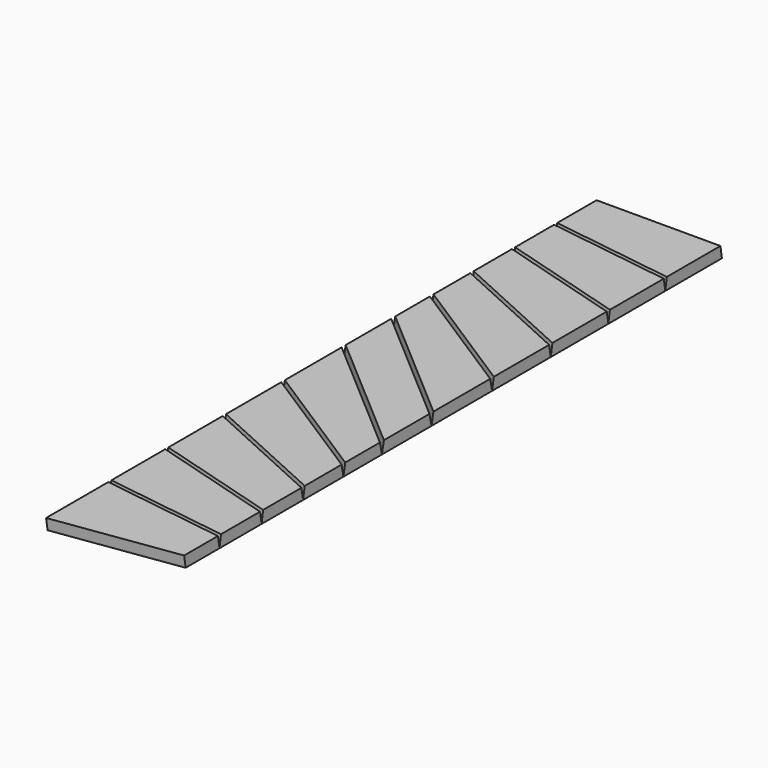
from build123d import *

# Parameters (mm, degrees)
F2_DEPTH    = 9.525
F3_DEPTH    = 9.525
F4_DEPTH    = 9.525
F5_DEPTH    = 9.525
F6_DEPTH    = 9.525
F7_DEPTH    = 9.525
F8_DEPTH    = 9.525
F9_DEPTH    = 9.525
F10_DEPTH   = 9.525
F11_DEPTH   = 9.525
F12_DEPTH   = 9.525
F13_SIZE2   = 1.550911
F13_SIZE    = 9.52499
F13_2_SIZE2 = 1.550911
F13_2_SIZE  = 9.52499
F14_SIZE2   = 1.550911
F14_SIZE    = 9.52499
F14_2_SIZE2 = 1.550911
F14_2_SIZE  = 9.52499
F15_SIZE2   = 1.550911
F15_SIZE    = 9.52499
F15_2_SIZE2 = 1.550911
F15_2_SIZE  = 9.52499
F16_SIZE2   = 1.550911
F16_SIZE    = 9.52499
F16_2_SIZE2 = 1.550911
F16_2_SIZE  = 9.52499
F17_SIZE2   = 1.550911
F17_SIZE    = 9.52499
F17_2_SIZE2 = 1.550911
F17_2_SIZE  = 9.52499
F18_SIZE2   = 1.550911
F18_SIZE    = 9.52499
F18_2_SIZE2 = 1.550911
F18_2_SIZE  = 9.52499
F19_SIZE2   = 1.550911
F19_SIZE    = 9.52499
F19_2_SIZE2 = 1.550911
F19_2_SIZE  = 9.52499
F20_SIZE2   = 1.550911
F20_SIZE    = 9.52499
F20_2_SIZE2 = 1.550911
F20_2_SIZE  = 9.52499
F21_SIZE2   = 1.550911
F21_SIZE    = 9.52499
F21_2_SIZE2 = 1.550911
F21_2_SIZE  = 9.52499
F22_SIZE2   = 1.550911
F22_SIZE    = 9.52499
F22_2_SIZE2 = 1.550911
F22_2_SIZE  = 9.52499
F23_SIZE2   = 1.550911
F23_SIZE    = 9.52499
F24_SIZE2   = 1.550911
F24_SIZE    = 9.52499


# Not quite as in the source:
# - a fillet or chamfer is up to 0.001 mm smaller than in the source, because OpenCascade refuses the exact size


with BuildPart() as f2:
    # F1 (on Top) → F2 (new body)
    with BuildSketch(Plane.XY):
        Polygon((50.8, 279.4), (-50.8, 279.4), (-50.8, 235.8864560812), (50.8, 221.3135439188), align=None)
    extrude(amount=F2_DEPTH)

    # F13 (size 9.525 and 1.5509205186 in the source; OpenCascade refuses exactly that, so slightly less here)
    f13_edges = [f2.edges().sort_by_distance(p)[0] for p in [
        (0, 228.6, 9.525),
    ]]
    f13_side = f2.faces().sort_by_distance((0, 228.6, 4.7625))[0]
    chamfer(f13_edges, length=F13_SIZE, length2=F13_SIZE2, reference=f13_side)

    # F13#2 (size 9.525 and 1.5509205186 in the source; OpenCascade refuses exactly that, so slightly less here)
    f13_2_edges = [f2.edges().sort_by_distance(p)[0] for p in [
        (0, 279.4, 9.525),
    ]]
    f13_2_side = f2.faces().sort_by_distance((0, 279.4, 4.7625))[0]
    chamfer(f13_2_edges, length=F13_2_SIZE, length2=F13_2_SIZE2, reference=f13_2_side)


with BuildPart() as f3:
    # F1 (on Top) → F3 (new body)
    with BuildSketch(Plane.XY):
        Polygon((50.8, 221.3135439188), (-50.8, 235.8864560812), (-50.8, 192.6790237109), (50.8, 162.9209762891), align=None)
    extrude(amount=F3_DEPTH)

    # F14 (size 9.525 and 1.5509205186 in the source; OpenCascade refuses exactly that, so slightly less here)
    f14_edges = [f3.edges().sort_by_distance(p)[0] for p in [
        (0, 228.6, 9.525),
    ]]
    f14_side = f3.faces().sort_by_distance((0, 228.6, 4.7625))[0]
    chamfer(f14_edges, length=F14_SIZE, length2=F14_SIZE2, reference=f14_side)

    # F14#2 (size 9.525 and 1.5509205186 in the source; OpenCascade refuses exactly that, so slightly less here)
    f14_2_edges = [f3.edges().sort_by_distance(p)[0] for p in [
        (0, 177.8, 9.525),
    ]]
    f14_2_side = f3.faces().sort_by_distance((0, 177.8, 4.7625))[0]
    chamfer(f14_2_edges, length=F14_2_SIZE, length2=F14_2_SIZE2, reference=f14_2_side)


with BuildPart() as f4:
    # F1 (on Top) → F4 (new body)
    with BuildSketch(Plane.XY):
        Polygon((50.8, 162.9209762891), (-50.8, 192.6790237109), (-50.8, 150.1375105152), (50.8, 103.8624894848), align=None)
    extrude(amount=F4_DEPTH)

    # F15 (size 9.525 and 1.5509205186 in the source; OpenCascade refuses exactly that, so slightly less here)
    f15_edges = [f4.edges().sort_by_distance(p)[0] for p in [
        (0, 177.8, 9.525),
    ]]
    f15_side = f4.faces().sort_by_distance((0, 177.8, 4.7625))[0]
    chamfer(f15_edges, length=F15_SIZE, length2=F15_SIZE2, reference=f15_side)

    # F15#2 (size 9.525 and 1.5509205186 in the source; OpenCascade refuses exactly that, so slightly less here)
    f15_2_edges = [f4.edges().sort_by_distance(p)[0] for p in [
        (0, 127, 9.525),
    ]]
    f15_2_side = f4.faces().sort_by_distance((0, 127, 4.7625))[0]
    chamfer(f15_2_edges, length=F15_2_SIZE, length2=F15_2_SIZE2, reference=f15_2_side)


with BuildPart() as f5:
    # F1 (on Top) → F5 (new body)
    with BuildSketch(Plane.XY):
        Polygon((50.8, 103.8624894848), (-50.8, 150.1375105152), (-50.8, 108.75045291), (50.8, 43.64954709), align=None)
    extrude(amount=F5_DEPTH)

    # F16 (size 9.525 and 1.5509205186 in the source; OpenCascade refuses exactly that, so slightly less here)
    f16_edges = [f5.edges().sort_by_distance(p)[0] for p in [
        (0, 127, 9.525),
    ]]
    f16_side = f5.faces().sort_by_distance((0, 127, 4.7625))[0]
    chamfer(f16_edges, length=F16_SIZE, length2=F16_SIZE2, reference=f16_side)

    # F16#2 (size 9.525 and 1.5509205186 in the source; OpenCascade refuses exactly that, so slightly less here)
    f16_2_edges = [f5.edges().sort_by_distance(p)[0] for p in [
        (0, 76.2, 9.525),
    ]]
    f16_2_side = f5.faces().sort_by_distance((0, 76.2, 4.7625))[0]
    chamfer(f16_2_edges, length=F16_2_SIZE, length2=F16_2_SIZE2, reference=f16_2_side)


with BuildPart() as f6:
    # F1 (on Top) → F6 (new body)
    with BuildSketch(Plane.XY):
        Polygon((50.8, 43.64954709), (-50.8, 108.75045291), (-50.8, 69.2687277608), (50.8, -18.4687277608), align=None)
    extrude(amount=F6_DEPTH)

    # F17 (size 9.525 and 1.5509205186 in the source; OpenCascade refuses exactly that, so slightly less here)
    f17_edges = [f6.edges().sort_by_distance(p)[0] for p in [
        (0, 25.4, 9.525),
    ]]
    f17_side = f6.faces().sort_by_distance((0, 25.4, 4.7625))[0]
    chamfer(f17_edges, length=F17_SIZE, length2=F17_SIZE2, reference=f17_side)

    # F17#2 (size 9.525 and 1.5509205186 in the source; OpenCascade refuses exactly that, so slightly less here)
    f17_2_edges = [f6.edges().sort_by_distance(p)[0] for p in [
        (0, 76.2, 9.525),
    ]]
    f17_2_side = f6.faces().sort_by_distance((0, 76.2, 4.7625))[0]
    chamfer(f17_2_edges, length=F17_2_SIZE, length2=F17_2_SIZE2, reference=f17_2_side)


with BuildPart() as f7:
    # F1 (on Top) → F7 (new body)
    with BuildSketch(Plane.XY):
        Polygon((50.8, -18.4687277608), (-50.8, 69.2687277608), (-50.8, 18.4687277609), (50.7999999999, -69.2687277608), align=None)
    extrude(amount=F7_DEPTH)

    # F18 (size 9.525 and 1.5509205186 in the source; OpenCascade refuses exactly that, so slightly less here)
    f18_edges = [f7.edges().sort_by_distance(p)[0] for p in [
        (0, 25.4, 9.525),
    ]]
    f18_side = f7.faces().sort_by_distance((0, 25.4, 4.7625))[0]
    chamfer(f18_edges, length=F18_SIZE, length2=F18_SIZE2, reference=f18_side)

    # F18#2 (size 9.525 and 1.5509205186 in the source; OpenCascade refuses exactly that, so slightly less here)
    f18_2_edges = [f7.edges().sort_by_distance(p)[0] for p in [
        (0, -25.4, 9.525),
    ]]
    f18_2_side = f7.faces().sort_by_distance((0, -25.4, 4.7625))[0]
    chamfer(f18_2_edges, length=F18_2_SIZE, length2=F18_2_SIZE2, reference=f18_2_side)


with BuildPart() as f8:
    # F1 (on Top) → F8 (new body)
    with BuildSketch(Plane.XY):
        Polygon((50.7999999999, -69.2687277608), (-50.8000000001, 18.4687277609), (-50.8, -43.64954709), (50.7999999999, -108.7504529099), align=None)
    extrude(amount=F8_DEPTH)

    # F19 (size 9.525 and 1.5509205186 in the source; OpenCascade refuses exactly that, so slightly less here)
    f19_edges = [f8.edges().sort_by_distance(p)[0] for p in [
        (0, -25.4, 9.525),
    ]]
    f19_side = f8.faces().sort_by_distance((0, -25.4, 4.7625))[0]
    chamfer(f19_edges, length=F19_SIZE, length2=F19_SIZE2, reference=f19_side)

    # F19#2 (size 9.525 and 1.5509205186 in the source; OpenCascade refuses exactly that, so slightly less here)
    f19_2_edges = [f8.edges().sort_by_distance(p)[0] for p in [
        (0, -76.2, 9.525),
    ]]
    f19_2_side = f8.faces().sort_by_distance((0, -76.2, 4.7625))[0]
    chamfer(f19_2_edges, length=F19_2_SIZE, length2=F19_2_SIZE2, reference=f19_2_side)


with BuildPart() as f9:
    # F1 (on Top) → F9 (new body)
    with BuildSketch(Plane.XY):
        Polygon((50.7999999999, -108.7504529099), (-50.8000000001, -43.64954709), (-50.8, -103.8624894848), (50.7999999999, -150.1375105152), align=None)
    extrude(amount=F9_DEPTH)

    # F20 (size 9.525 and 1.5509205186 in the source; OpenCascade refuses exactly that, so slightly less here)
    f20_edges = [f9.edges().sort_by_distance(p)[0] for p in [
        (0, -76.2, 9.525),
    ]]
    f20_side = f9.faces().sort_by_distance((0, -76.2, 4.7625))[0]
    chamfer(f20_edges, length=F20_SIZE, length2=F20_SIZE2, reference=f20_side)

    # F20#2 (size 9.525 and 1.5509205186 in the source; OpenCascade refuses exactly that, so slightly less here)
    f20_2_edges = [f9.edges().sort_by_distance(p)[0] for p in [
        (0, -127, 9.525),
    ]]
    f20_2_side = f9.faces().sort_by_distance((0, -127, 4.7625))[0]
    chamfer(f20_2_edges, length=F20_2_SIZE, length2=F20_2_SIZE2, reference=f20_2_side)


with BuildPart() as f10:
    # F1 (on Top) → F10 (new body)
    with BuildSketch(Plane.XY):
        Polygon((50.7999999999, -150.1375105152), (-50.8000000001, -103.8624894848), (-50.8, -162.9209762891), (50.7999999999, -192.6790237109), align=None)
    extrude(amount=F10_DEPTH)

    # F21 (size 9.525 and 1.5509205186 in the source; OpenCascade refuses exactly that, so slightly less here)
    f21_edges = [f10.edges().sort_by_distance(p)[0] for p in [
        (0, -127, 9.525),
    ]]
    f21_side = f10.faces().sort_by_distance((0, -127, 4.7625))[0]
    chamfer(f21_edges, length=F21_SIZE, length2=F21_SIZE2, reference=f21_side)

    # F21#2 (size 9.525 and 1.5509205186 in the source; OpenCascade refuses exactly that, so slightly less here)
    f21_2_edges = [f10.edges().sort_by_distance(p)[0] for p in [
        (0, -177.8, 9.525),
    ]]
    f21_2_side = f10.faces().sort_by_distance((0, -177.8, 4.7625))[0]
    chamfer(f21_2_edges, length=F21_2_SIZE, length2=F21_2_SIZE2, reference=f21_2_side)


with BuildPart() as f11:
    # F1 (on Top) → F11 (new body)
    with BuildSketch(Plane.XY):
        Polygon((50.7999999999, -192.6790237109), (-50.8000000001, -162.9209762891), (-50.8, -221.3135439188), (50.7999999999, -235.8864560811), align=None)
    extrude(amount=F11_DEPTH)

    # F22 (size 9.525 and 1.5509205186 in the source; OpenCascade refuses exactly that, so slightly less here)
    f22_edges = [f11.edges().sort_by_distance(p)[0] for p in [
        (0, -177.8, 9.525),
    ]]
    f22_side = f11.faces().sort_by_distance((0, -177.8, 4.7625))[0]
    chamfer(f22_edges, length=F22_SIZE, length2=F22_SIZE2, reference=f22_side)

    # F22#2 (size 9.525 and 1.5509205186 in the source; OpenCascade refuses exactly that, so slightly less here)
    f22_2_edges = [f11.edges().sort_by_distance(p)[0] for p in [
        (0, -228.6, 9.525),
    ]]
    f22_2_side = f11.faces().sort_by_distance((0, -228.6, 4.7625))[0]
    chamfer(f22_2_edges, length=F22_2_SIZE, length2=F22_2_SIZE2, reference=f22_2_side)


with BuildPart() as f12:
    # F1 (on Top) → F12 (new body)
    with BuildSketch(Plane.XY):
        Polygon((50.7999999999, -235.8864560811), (-50.8000000001, -221.3135439188), (-50.8, -279.4), (-50.8, -286.6864560812), (50.8, -272.1135439188), align=None)
    extrude(amount=F12_DEPTH)

    # F23 (size 9.525 and 1.5509205186 in the source; OpenCascade refuses exactly that, so slightly less here)
    f23_edges = [f12.edges().sort_by_distance(p)[0] for p in [
        (0, -228.6, 9.525),
    ]]
    f23_side = f12.faces().sort_by_distance((0, -228.6, 4.7625))[0]
    chamfer(f23_edges, length=F23_SIZE, length2=F23_SIZE2, reference=f23_side)

    # F24 (size 9.525 and 1.5509205186 in the source; OpenCascade refuses exactly that, so slightly less here)
    f24_edges = [f12.edges().sort_by_distance(p)[0] for p in [
        (0, -279.4, 0),
    ]]
    f24_side = f12.faces().sort_by_distance((0, -279.4, 4.7625))[0]
    chamfer(f24_edges, length=F24_SIZE, length2=F24_SIZE2, reference=f24_side)


solid = Compound([f2.part, f3.part, f4.part, f5.part, f6.part, f7.part, f8.part, f9.part, f10.part, f11.part, f12.part])
